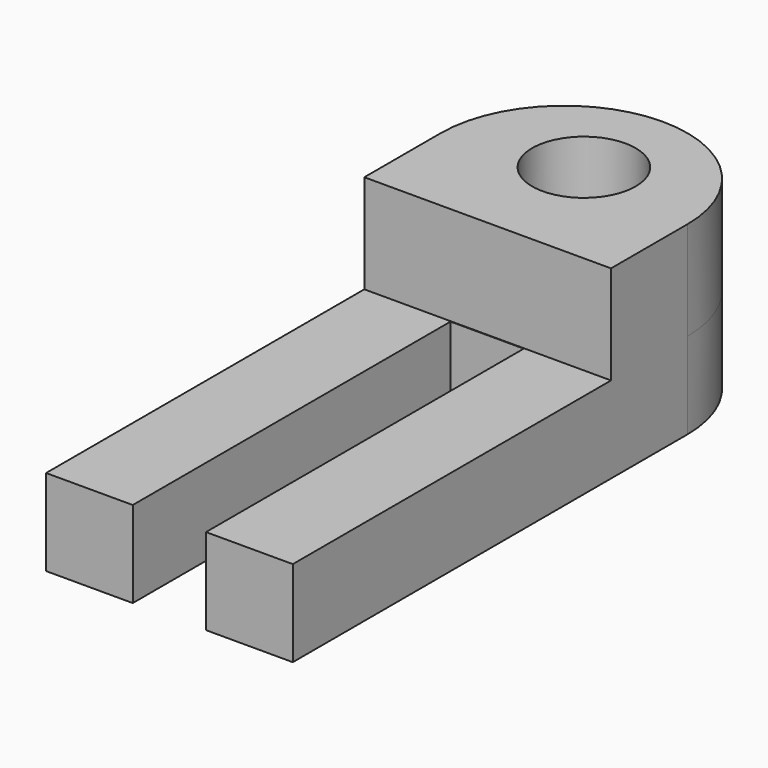
from build123d import *

# Parameters (mm, degrees)
F0_R     = 2.1
F1_DEPTH = 3.5
F2_R     = 4.99999
F3_R     = 2.1
F4_DEPTH = 4


# Not quite as in the source:
# - a fillet or chamfer is up to 0.001 mm smaller than in the source, because OpenCascade refuses the exact size
# - ends of sketch curves that miss each other by under 0.0002 mm in the source are joined


with BuildPart() as f1:
    # F0 (on Top) → F1 (new body)
    with BuildSketch(Plane.XY):
        Polygon((1.4820488868, -12.5), (5, -12.5), (5, 12.5), (-5, 12.5), (-5, -12.5), (-1.4866787242, -12.5), (-1.4866787242, 3.6), (1.4820488868, 3.6), align=None)
        with Locations((0, 8.5)):
            Circle(F0_R, mode=Mode.SUBTRACT)
    extrude(amount=F1_DEPTH)

    # F2 (radius 5 in the source; OpenCascade refuses exactly that, so slightly less here)
    f2_edges = [f1.edges().sort_by_distance(p)[0] for p in [
        (-5, 12.5, 1.75),
        (5, 12.5, 1.75),
    ]]
    fillet(f2_edges, radius=F2_R)

    # F3 (on face) → F4 (join)
    with BuildSketch(Plane.XY.offset(3.5)):
        with BuildLine():
            Line((-5, 3.6241896451), (0, 3.6241896451))
            Line((0, 3.6241896451), (5, 3.6241896451))
            Line((5, 3.6241896451), (5, 7.50001))
            ThreePointArc((5, 7.50001), (3.5355368349, 11.0355368349), (1e-05, 12.5))
            ThreePointArc((1e-05, 12.5), (-3.5355368349, 11.0355368349), (-5, 7.50001))
            Line((-5, 7.50001), (-5, 3.6241896451))
        make_face()
        with Locations((0, 8.5)):
            Circle(F3_R, mode=Mode.SUBTRACT)
    extrude(amount=F4_DEPTH)


solid = f1.part
